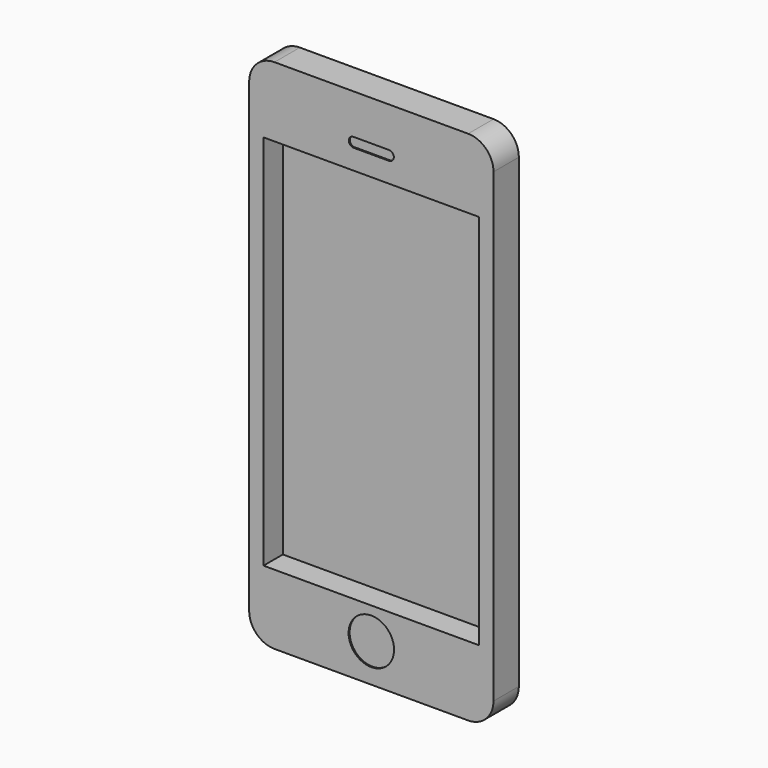
from build123d import *

# Parameters (mm, degrees)
F0_W     = 51.7
F0_H     = 90.39
F0_W_2   = 10.8
F0_H_2   = 2.3
F1_DEPTH = 7.6
F2_R     = 6.07
F3_DEPTH = 1.8
F4_R     = 1.14999
F5_DEPTH = 7.3
F6_DEPTH = 7.3


# Not quite as in the source:
# - a fillet or chamfer is up to 0.001 mm smaller than in the source, because OpenCascade refuses the exact size


with BuildPart() as f1:
    # F0 (on Front) → F1 (new body)
    with BuildSketch(Plane.XZ):
        Polygon((0, -61.915), (29.285, -61.915), (29.285, 61.915), (-29.285, 61.915), (-29.285, -61.915), align=None)
        with BuildLine():
            ThreePointArc((5.45, -52.765), (3.8537319575, -56.6187319575), (0, -58.215))
            ThreePointArc((0, -58.215), (-3.8537319575, -48.9112680425), (5.45, -52.765))
        make_face(mode=Mode.SUBTRACT)
        Rectangle(F0_W, F0_H, mode=Mode.SUBTRACT)
        with Locations((0, 51.165)):
            Rectangle(F0_W_2, F0_H_2, mode=Mode.SUBTRACT)
    extrude(amount=F1_DEPTH)

    # F2
    f2_edges = [f1.edges().sort_by_distance(p)[0] for p in [
        (-29.285, -3.8, 61.915),
        (29.285, -3.8, 61.915),
        (-29.285, -3.8, -61.915),
        (29.285, -3.8, -61.915),
    ]]
    fillet(f2_edges, radius=F2_R)

    # F0 (on Front) → F3 (join)
    with BuildSketch(Plane.XZ):
        Rectangle(F0_W, F0_H)
    extrude(amount=F3_DEPTH)

    # F4 (radius 1.15 in the source; OpenCascade refuses exactly that, so slightly less here)
    f4_edges = [f1.edges().sort_by_distance(p)[0] for p in [
        (-5.4, -3.8, 52.315),
        (5.4, -3.8, 52.315),
        (5.4, -3.8, 50.015),
        (-5.4, -3.8, 50.015),
    ]]
    fillet(f4_edges, radius=F4_R)

    # F0 (on Front) → F5 (join)
    with BuildSketch(Plane.XZ):
        with Locations((0, 51.165)):
            Rectangle(F0_W_2, F0_H_2)
    extrude(amount=F5_DEPTH)

    # F0 (on Front) → F6 (join)
    with BuildSketch(Plane.XZ):
        with BuildLine():
            ThreePointArc((5.45, -52.765), (-3.8537319575, -48.9112680425), (0, -58.215))
            ThreePointArc((0, -58.215), (3.8537319575, -56.6187319575), (5.45, -52.765))
        make_face()
    extrude(amount=F6_DEPTH)


solid = f1.part
